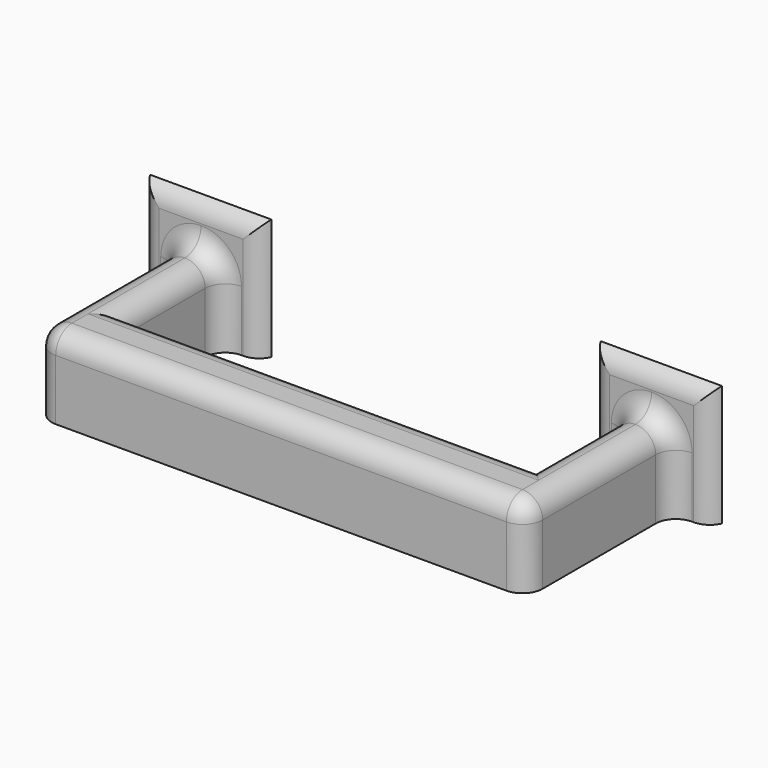
from build123d import *

# Parameters (mm, degrees)
F0_W        = 101.6
F0_H        = 15
F1_DEPTH    = 20
F2_W        = 30
F2_H        = 30
F3_DEPTH    = 3
F4_R        = 4.99999
F5_T1_DEPTH = 52.9128784748
F5_T3_DEPTH = 52.9128784748
F5_T5_DEPTH = 52.9128784748


# Not quite as in the source:
# - a fillet or chamfer that OpenCascade refuses, or shapes differently, is made with other operations: its cross-section is extruded or revolved along the edge and cut away or added
# - a fillet or chamfer is up to 0.001 mm smaller than in the source, because OpenCascade refuses the exact size
# - a feature of the source that left no trace in its solid (it failed there, or was rolled back) is left out


with BuildPart() as f1:
    # F0 (on Top) → F1 (new body)
    with BuildSketch(Plane.XY):
        Rectangle(F0_W, F0_H)
        Polygon((50.8, 7.5), (50.8, -7.5), (60.8, -7.5), (60.8, 37.5), (50.8, 37.5), align=None)
        Polygon((-60.8, -7.5), (-50.8, -7.5), (-50.8, 7.5), (-50.8, 37.5), (-60.8, 37.5), align=None)
    extrude(amount=F1_DEPTH)

    # F2 (on face) → F3 (join)
    with BuildSketch(Plane(origin=(0, 37.5, 0), x_dir=(-1, 0, 0), z_dir=(0, 1, 0))):
        with Locations((-55.8, 15)):
            Rectangle(F2_W, F2_H)
        with Locations((55.8, 15)):
            Rectangle(F2_W, F2_H)
    extrude(amount=F3_DEPTH)

    # F4 (radius 5 in the source; OpenCascade refuses exactly that, so slightly less here)
    f4_edges = [f1.edges().sort_by_distance(p)[0] for p in [
        (-55.8, 37.5, 20),
        (-50.8, 37.5, 10),
        (-60.8, 37.5, 10),
        (-60.8, -7.5, 10),
        (60.8, -7.5, 10),
        (60.8, 37.5, 10),
        (55.8, 37.5, 20),
        (50.8, 37.5, 10),
        (60.8, 15, 20),
        (50.8, 22.5, 20),
        (0, 7.5, 20),
        (-50.8, 22.5, 20),
        (-60.8, 15, 20),
        (0, -7.5, 20),
    ]]
    fillet(f4_edges, radius=F4_R)

    # F5: fillet of radius 5 on 6 edges, made by hand

    # F5_s2 → F5_t1 (cut)
    with BuildSketch(Plane.YZ.offset(-82.2564392374)):
        with BuildLine():
            ThreePointArc((37.5, 25.417424305), (38.3166998673, 28.1560370926), (40.5, 30))
            Line((40.5, 30), (37.5, 30))
            Line((37.5, 30), (37.5, 25.417424305))
        make_face()
    extrude(amount=F5_T1_DEPTH, mode=Mode.SUBTRACT)

    # F5_s4 → F5_t3 (cut)
    with BuildSketch(Plane.XY.offset(-11.4564392374)):
        with BuildLine():
            ThreePointArc((-66.217424305, 37.5), (-68.9560370926, 38.3166998673), (-70.8, 40.5))
            Line((-70.8, 40.5), (-70.8, 37.5))
            Line((-70.8, 37.5), (-66.217424305, 37.5))
        make_face()
        with BuildLine():
            ThreePointArc((-45.382575695, 37.5), (-42.6439629074, 38.3166998673), (-40.8, 40.5))
            Line((-40.8, 40.5), (-40.8, 37.5))
            Line((-40.8, 37.5), (-45.382575695, 37.5))
        make_face()
        with BuildLine():
            ThreePointArc((45.382575695, 37.5), (42.6439629074, 38.3166998673), (40.8, 40.5))
            Line((40.8, 40.5), (40.8, 37.5))
            Line((40.8, 37.5), (45.382575695, 37.5))
        make_face()
        with BuildLine():
            ThreePointArc((66.217424305, 37.5), (68.9560370926, 38.3166998673), (70.8, 40.5))
            Line((70.8, 40.5), (70.8, 37.5))
            Line((70.8, 37.5), (66.217424305, 37.5))
        make_face()
    extrude(amount=F5_T3_DEPTH, mode=Mode.SUBTRACT)

    # F5_s6 → F5_t5 (cut)
    with BuildSketch(Plane.YZ.offset(29.3435607626)):
        with BuildLine():
            ThreePointArc((37.5, 25.417424305), (38.3166998673, 28.1560370926), (40.5, 30))
            Line((40.5, 30), (37.5, 30))
            Line((37.5, 30), (37.5, 25.417424305))
        make_face()
    extrude(amount=F5_T5_DEPTH, mode=Mode.SUBTRACT)


solid = f1.part
